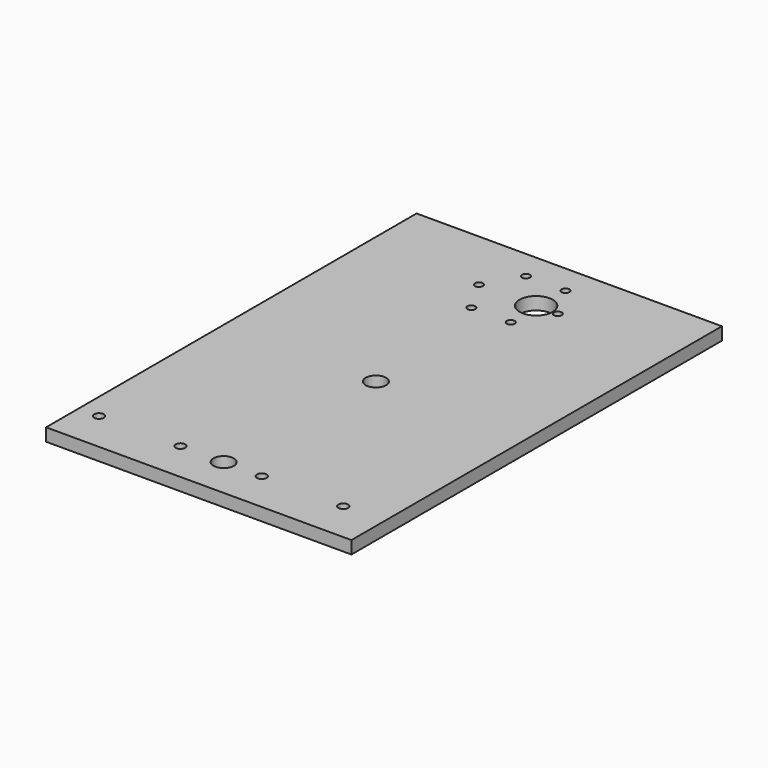
from build123d import *

# Parameters (mm, degrees)
F0_W     = 120
F0_H     = 132
F0_R     = 1.9
F0_R_2   = 4
F0_H_2   = 50
F0_R_3   = 1.55
F0_R_4   = 6.5
F1_DEPTH = 5
F2_R     = 4
F3_DEPTH = 25


# Not quite as in the source:
# - a feature names something its author has since deleted; it is built from what else it names


with BuildPart() as f1:
    # F0 (on Top) → F1 (new body)
    with BuildSketch(Plane.XY):
        Rectangle(F0_W, F0_H)
        with Locations((-52, -50)):
            Circle(F0_R, mode=Mode.SUBTRACT)
        with Locations((-20, -50)):
            Circle(F0_R, mode=Mode.SUBTRACT)
        with Locations((-3, -50)):
            Circle(F0_R_2, mode=Mode.SUBTRACT)
        with Locations((12, -50)):
            Circle(F0_R, mode=Mode.SUBTRACT)
        with Locations((44, -50)):
            Circle(F0_R, mode=Mode.SUBTRACT)
        with Locations((0, 91)):
            Rectangle(F0_W, F0_H_2)
        with Locations((-15.5, 91)):
            Circle(F0_R_3, mode=Mode.SUBTRACT)
        with Locations((-7.75, 77.5766062413)):
            Circle(F0_R_3, mode=Mode.SUBTRACT)
        with Locations((-7.75, 104.4233937587)):
            Circle(F0_R_3, mode=Mode.SUBTRACT)
        with Locations((7.75, 77.5766062413)):
            Circle(F0_R_3, mode=Mode.SUBTRACT)
        with Locations((6.9857463241, 91)):
            Circle(F0_R_4, mode=Mode.SUBTRACT)
        with Locations((15.5, 91)):
            Circle(F0_R_3, mode=Mode.SUBTRACT)
        with Locations((7.75, 104.4233937587)):
            Circle(F0_R_3, mode=Mode.SUBTRACT)
    extrude(amount=F1_DEPTH)

    # F2 (on face) → F3 (cut)
    with BuildSketch(Plane.XY.offset(5)):
        with Locations((0, 21)):
            Circle(F2_R)
    extrude(amount=-F3_DEPTH, mode=Mode.SUBTRACT)


solid = f1.part
